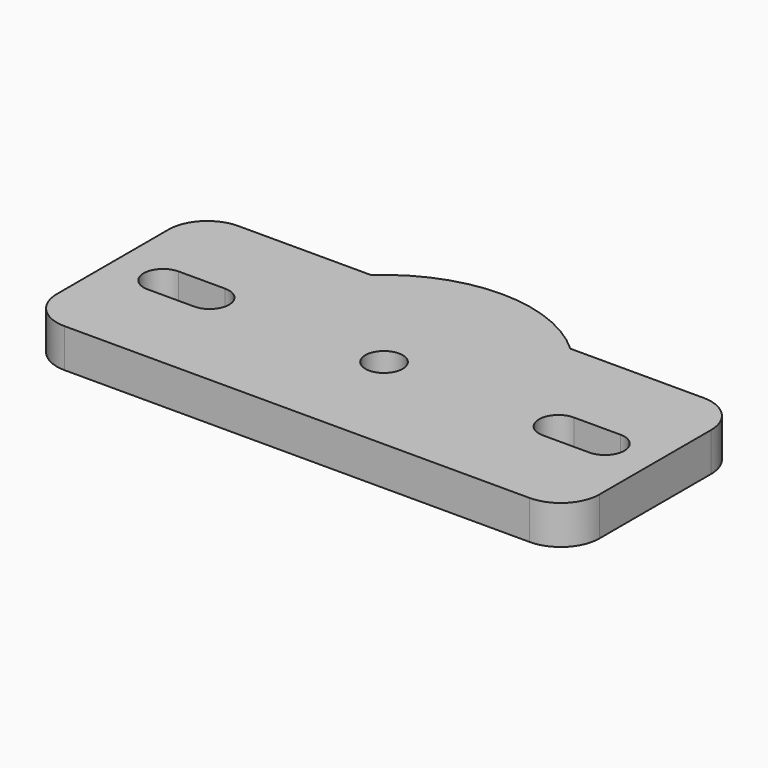
from build123d import *

# Parameters (mm, degrees)
F0_R     = 2.4
F0_W     = 18
F0_H     = 4
F1_DEPTH = 5


# Not quite as in the source:
# - ends of sketch curves that miss each other by under 0.0002 mm in the source are joined


with BuildPart() as f1:
    # F0 (on Top) → F1 (new body)
    with BuildSketch(Plane.XY):
        with BuildLine():
            Line((-12.8452325787, 14), (-30, 14))
            ThreePointArc((-30, 14), (-33.5355339059, 12.5355339059), (-35, 9))
            Line((-35, 9), (-35, -9))
            ThreePointArc((-35, -9), (-33.5355339059, -12.5355339059), (-30, -14))
            Line((-30, -14), (-12.8452325787, -14))
            ThreePointArc((-12.8452325787, -14), (-19, 0), (-12.8452325787, 14))
        make_face()
        with BuildLine():
            ThreePointArc((-28.5, -2.5), (-31, 0), (-28.5, 2.5))
            Line((-28.5, 2.5), (-22.5, 2.5))
            ThreePointArc((-22.5, 2.5), (-20.7249314431, 1.7717582393), (-19.9886980778, 0))
            ThreePointArc((-19.9886980778, 0), (-20.724931484, -1.77175828), (-22.5, -2.4999744532))
            Line((-22.5, -2.4999744532), (-28.5, -2.5))
        make_face(mode=Mode.SUBTRACT)
        with BuildLine():
            Line((12.8452325787, 14), (-12.8452325787, 14))
            ThreePointArc((-12.8452325787, 14), (-19, 0), (-12.8452325787, -14))
            add(Edge.make_bspline(
                [(-9, -10), (-10.2817441929, -11.3333333333), (-11.5634883858, -12.6666666667), (-12.8452325787, -14)],
                knots=[0, 0, 0, 0, 5.5484965156, 5.5484965156, 5.5484965156, 5.5484965156], degree=3))
            Line((-9, -10), (9, -10))
            add(Edge.make_bspline(
                [(9, -10), (10.2817441929, -11.3333333333), (11.5634883858, -12.6666666667), (12.8452325787, -14)],
                knots=[0, 0, 0, 0, 5.5484965156, 5.5484965156, 5.5484965156, 5.5484965156], degree=3))
            ThreePointArc((12.8452325787, -14), (17.393381198, -7.6465868531), (19, 0))
            ThreePointArc((19, 0), (17.393381198, 7.6465868531), (12.8452325787, 14))
        make_face()
        Circle(F0_R, mode=Mode.SUBTRACT)
        with BuildLine():
            ThreePointArc((12.8452325787, 14), (0, 19), (-12.8452325787, 14))
            Line((-12.8452325787, 14), (12.8452325787, 14))
        make_face()
        with BuildLine():
            Line((30, 14), (12.8452325787, 14))
            ThreePointArc((12.8452325787, 14), (17.393381198, 7.6465868531), (19, 0))
            ThreePointArc((19, 0), (17.393381198, -7.6465868531), (12.8452325787, -14))
            Line((12.8452325787, -14), (30, -14))
            ThreePointArc((30, -14), (33.5355339059, -12.5355339059), (35, -9))
            Line((35, -9), (35, 9))
            ThreePointArc((35, 9), (33.5355339059, 12.5355339059), (30, 14))
        make_face()
        with BuildLine():
            ThreePointArc((22.5, -2.5), (20, 0), (22.5, 2.5))
            Line((22.5, 2.5), (28.5, 2.5))
            ThreePointArc((28.5, 2.5), (30.267766953, 1.767766953), (31, 0))
            ThreePointArc((31, 0), (30.267766953, -1.767766953), (28.5, -2.5))
            Line((28.5, -2.5), (22.5, -2.5))
        make_face(mode=Mode.SUBTRACT)
        with Locations((0, -12)):
            Rectangle(F0_W, F0_H)
        with BuildLine():
            add(Edge.make_bspline(
                [(-9, -10), (-10.2817441929, -11.3333333333), (-11.5634883858, -12.6666666667), (-12.8452325787, -14)],
                knots=[0, 0, 0, 0, 5.5484965156, 5.5484965156, 5.5484965156, 5.5484965156], degree=3))
            Line((-12.8452325787, -14), (-9, -14))
            Line((-9, -14), (-9, -10))
        make_face()
        with BuildLine():
            Line((9, -14), (12.8452325787, -14))
            add(Edge.make_bspline(
                [(9, -10), (10.2817441929, -11.3333333333), (11.5634883858, -12.6666666667), (12.8452325787, -14)],
                knots=[0, 0, 0, 0, 5.5484965156, 5.5484965156, 5.5484965156, 5.5484965156], degree=3))
            Line((9, -10), (9, -14))
        make_face()
    extrude(amount=F1_DEPTH)


solid = f1.part
